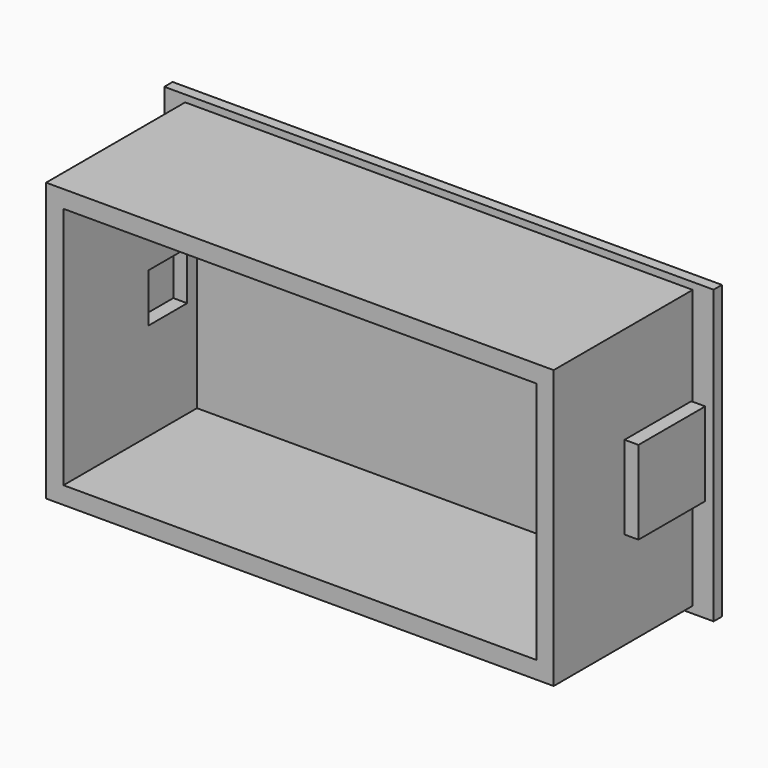
from build123d import *

# Parameters (mm, degrees)
F0_W        = 73
F0_H        = 40
F1_DEPTH    = 26.5
F0_W_2      = 79
F0_H_2      = 42
F2_DEPTH    = 1.5
F3_W        = 12
F3_H        = 12
F4_DEPTH    = 2
F5_W        = 12
F5_H        = 12
F6_DEPTH    = 2
F7_T        = 2.5
F7_T3_DEPTH = 78
F7_T5_DEPTH = 45
F7_T7_DEPTH = 17
F7_T9_DEPTH = 17


# Not quite as in the source:
# - a shell that OpenCascade refuses in one call is made with other operations: the cavity is built on its own and cut out


with BuildPart() as f1:
    # F0 (on Front) → F1 (new body)
    with BuildSketch(Plane.XZ):
        Rectangle(F0_W, F0_H)
    extrude(amount=F1_DEPTH)

    # F0 (on Front) → F2 (join)
    with BuildSketch(Plane.XZ):
        Rectangle(F0_W_2, F0_H_2)
        Rectangle(F0_W, F0_H, mode=Mode.SUBTRACT)
    extrude(amount=F2_DEPTH)

    # F3 (on face) → F4 (join)
    with BuildSketch(Plane(origin=(-36.5, 0, 0), x_dir=(0, -1, 0), z_dir=(-1, 0, 0))):
        with Locations((7.75, 0)):
            Rectangle(F3_W, F3_H)
    extrude(amount=F4_DEPTH)

    # F5 (on face) → F6 (join)
    with BuildSketch(Plane.YZ.offset(36.5)):
        with Locations((-7.75, 0)):
            Rectangle(F5_W, F5_H)
    extrude(amount=F6_DEPTH)

    # F7: shell of thickness 2.5, made by hand


with BuildPart() as f7_core1:
    # F7_t2: copy of F1
    add(f1.part)

    # the walls: a layer under each face that stays
    f7_faces = [f7_core1.faces().sort_by_distance(p)[0] for p in [
        (0, -14, -20),
        (-36.8666666667, -1.5, -19.6),
        (36.5, -14, 0),
        (-36.5, -14, 0),
        (0, -0.75, -21),
        (39.5, -0.75, 0),
        (0, -0.75, 21),
        (-39.5, -0.75, 0),
        (0, -14, 20),
        (37.5, -13.75, 0),
        (37.5, -7.75, 6),
        (37.5, -1.75, 0),
        (37.5, -7.75, -6),
        (-37.5, -1.75, 0),
        (-37.5, -7.75, 6),
        (-37.5, -13.75, 0),
        (-37.5, -7.75, -6),
        (0, 0, 0),
        (38.5, -7.75, 0),
        (-38.5, -7.75, 0),
    ]]
    thicken(f7_faces, amount=-F7_T, mode=Mode.SUBTRACT)

    # F7_s4 → F7_t3 (cut)
    with BuildSketch(Plane.YZ.offset(-39)):
        Polygon((-1.525, -20.025), (-1.5, -17.5), (1, -17.5), (1, -20), align=None)
        Polygon((-1.525, 20.025), (1, 20), (1, 17.5), (-1.5, 17.5), align=None)
    extrude(amount=F7_T3_DEPTH, mode=Mode.SUBTRACT)

    # F7_s6 → F7_t5 (cut)
    with BuildSketch(Plane.XY.offset(-22.5)):
        Polygon((36.525, -1.525), (36.5, 1), (34, 1), (34, -1.5), align=None)
        Polygon((-36.525, -1.525), (-36.5, 1), (-34, 1), (-34, -1.5), align=None)
    extrude(amount=F7_T5_DEPTH, mode=Mode.SUBTRACT)

    # F7_s8 → F7_t7 (cut)
    with BuildSketch(Plane.XY.offset(-8.5)):
        Polygon((36.525, -13.775), (34, -13.75), (34, -11.25), (36.5, -11.25), align=None)
        Polygon((36.525, -1.725), (34, -1.75), (34, -4.25), (36.5, -4.25), align=None)
        Polygon((-36.525, -1.725), (-34, -1.75), (-34, -4.25), (-36.5, -4.25), align=None)
        Polygon((-36.525, -13.775), (-34, -13.75), (-34, -11.25), (-36.5, -11.25), align=None)
    extrude(amount=F7_T7_DEPTH, mode=Mode.SUBTRACT)

    # F7_s10 → F7_t9 (cut)
    with BuildSketch(Plane.XZ.offset(-0.75)):
        Polygon((36.525, 6.025), (34, 6), (34, 3.5), (36.5, 3.5), align=None)
        Polygon((36.525, -6.025), (34, -6), (34, -3.5), (36.5, -3.5), align=None)
        Polygon((-36.525, 6.025), (-34, 6), (-34, 3.5), (-36.5, 3.5), align=None)
        Polygon((-36.525, -6.025), (-34, -6), (-34, -3.5), (-36.5, -3.5), align=None)
    extrude(amount=F7_T9_DEPTH, mode=Mode.SUBTRACT)


with BuildPart() as f1_1:
    add(f1.part)

    # what is left inside the walls is the cavity
    f7_cavity = [f7_core1.part.solids().sort_by_distance(p)[0] for p in [
        (0, -2.525, -5.833333),
    ]]
    add(f7_cavity, mode=Mode.SUBTRACT)


solid = f1_1.part
